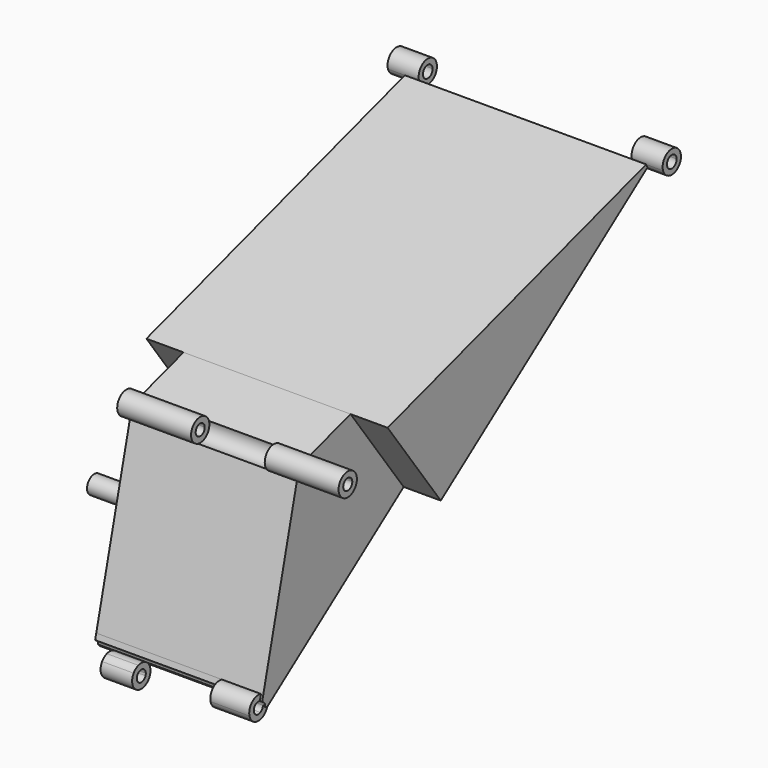
from build123d import *
from build123d import SkipClean  # not in build123d's __all__

# Parameters (mm, degrees)
F1_START = -16.65
F1_DEPTH = 79.6
F2_START = -37.25
F2_DEPTH = 34
F3_START = -114.75
F3_DEPTH = 33.5
F4_START = 62.75
F4_DEPTH = 79.6
F5_START = 45.55
F5_DEPTH = 42
F0_R     = 9.8
F6_DEPTH = 150
F8_DEPTH = 90
F9_DEPTH = 130


# Not quite as in the source:
# - after a boolean that leaves OpenCascade's solid faulty, fix() repairs it


with BuildPart() as f1:
    # F0 (on Right) → F1 (new body)
    with BuildSketch(Plane.YZ.offset(F1_START)):
        with BuildLine():
            Line((-18.1152243821, 20.3958344616), (-12.1555414908, 22.2498694633))
            ThreePointArc((-12.1555414908, 22.2498694633), (-32.9276080285, 27.0414189792), (-26.8836398395, 6.5986172255))
            Line((-26.8836398395, 6.5986172255), (-25.3948918397, 12.6598790865))
            ThreePointArc((-25.3948918397, 12.6598790865), (-28.3822482179, 22.7641569875), (-18.1152243821, 20.3958344616))
        make_face()
        with BuildLine():
            ThreePointArc((-26.8836398395, 6.5986172255), (-16.3247484731, 8.8719395429), (-11.5984598892, 18.5838074099))
            ThreePointArc((-11.5984598892, 18.5838074099), (-11.7385251038, 20.4378806886), (-12.1555414908, 22.2498694633))
            Line((-12.1555414908, 22.2498694633), (-18.1152243821, 20.3958344616))
            ThreePointArc((-18.1152243821, 20.3958344616), (-17.9091054013, 19.5002215043), (-17.8398752699, 18.5838074099))
            ThreePointArc((-17.8398752699, 18.5838074099), (-20.1759412293, 13.7835156961), (-25.3948918397, 12.6598790865))
            Line((-25.3948918397, 12.6598790865), (-26.8836398395, 6.5986172255))
        make_face()
    extrude(amount=-F1_DEPTH)



with BuildPart() as f2:
    # F0 (on Right) → F2 (new body)
    with BuildSketch(Plane.YZ.offset(F2_START)):
        with BuildLine():
            Line((-72.6551036638, -196.2316651642), (-67.6112595051, -192.5554031964))
            ThreePointArc((-67.6112595051, -192.5554031964), (-68.6065299554, -191.356834242), (-69.7448706932, -190.2932031158))
            ThreePointArc((-69.7448706932, -190.2932031158), (-70.6550390715, -193.4685207262), (-73.0869940433, -195.7038380233))
            ThreePointArc((-73.0869940433, -195.7038380233), (-72.8636664269, -195.9617109817), (-72.6551036638, -196.2316651642))
        make_face()
        with BuildLine():
            ThreePointArc((-69.7448706932, -190.2932031158), (-72.0550616531, -188.7913185641), (-74.6409019404, -187.8394417408))
            Line((-74.6409019404, -187.8394417408), (-76.1296499401, -193.9007036018))
            ThreePointArc((-76.1296499401, -193.9007036018), (-74.4747709929, -194.5769133854), (-73.0869940433, -195.7038380233))
            ThreePointArc((-73.0869940433, -195.7038380233), (-70.6550390715, -193.4685207262), (-69.7448706932, -190.2932031158))
        make_face()
        with BuildLine():
            Line((-76.1296499401, -193.9007036018), (-74.6409019404, -187.8394417408))
            ThreePointArc((-74.6409019404, -187.8394417408), (-78.1243753606, -187.4950233364), (-81.5644298108, -188.1425080744))
            ThreePointArc((-81.5644298108, -188.1425080744), (-81.831132306, -191.4349111758), (-80.3424675585, -194.3836271121))
            ThreePointArc((-80.3424675585, -194.3836271121), (-78.2793719358, -193.7643196914), (-76.1296499401, -193.9007036018))
        make_face()
        with BuildLine():
            ThreePointArc((-81.5644298108, -188.1425080744), (-85.124263165, -190.0540118898), (-87.8759224883, -193.012834513))
            ThreePointArc((-87.8759224883, -193.012834513), (-86.3429062121, -196.7512996317), (-83.6845909086, -199.7942620195))
            ThreePointArc((-83.6845909086, -199.7942620195), (-82.7744225302, -196.6189444092), (-80.3424675585, -194.3836271121))
            ThreePointArc((-80.3424675585, -194.3836271121), (-81.831132306, -191.4349111758), (-81.5644298108, -188.1425080744))
        make_face()
        with BuildLine():
            ThreePointArc((-83.6845909086, -199.7942620195), (-86.3429062121, -196.7512996317), (-87.8759224883, -193.012834513))
            ThreePointArc((-87.8759224883, -193.012834513), (-81.1414817132, -211.6423981781), (-65.2432511293, -199.8246319252))
            ThreePointArc((-65.2432511293, -199.8246319252), (-65.3210684593, -198.4409063564), (-65.5535391134, -197.0746306224))
            ThreePointArc((-65.5535391134, -197.0746306224), (-68.3051984367, -200.0334532455), (-71.865031791, -201.944957061))
            ThreePointArc((-71.865031791, -201.944957061), (-78.6766955162, -205.8260878027), (-83.6845909086, -199.7942620195))
        make_face()
        with BuildLine():
            ThreePointArc((-65.5535391134, -197.0746306224), (-66.3527593839, -194.7104559496), (-67.6112595051, -192.5554031964))
            Line((-67.6112595051, -192.5554031964), (-72.6551036638, -196.2316651642))
            ThreePointArc((-72.6551036638, -196.2316651642), (-71.7846521409, -197.9352316714), (-71.48466651, -199.8246319252))
            ThreePointArc((-71.48466651, -199.8246319252), (-71.5805107914, -200.9017178582), (-71.865031791, -201.944957061))
            ThreePointArc((-71.865031791, -201.944957061), (-68.3051984367, -200.0334532455), (-65.5535391134, -197.0746306224))
        make_face()
    extrude(amount=-F2_DEPTH)


with BuildPart() as f3:
    # F0 (on Right) → F3 (new body)
    with BuildSketch(Plane.YZ.offset(F3_START)):
        with BuildLine():
            Line((399.0634596914, 150.1785588691), (393.4857211205, 148.4433453134))
            ThreePointArc((393.4857211205, 148.4433453134), (394.2430188732, 146.5672949475), (395.2966478948, 144.840178638))
            Line((395.2966478948, 144.840178638), (400.0172420308, 148.2808362281))
            ThreePointArc((400.0172420308, 148.2808362281), (399.4623147045, 149.1904771133), (399.0634596914, 150.1785588691))
        make_face()
        with BuildLine():
            ThreePointArc((417.6114702803, 152.1094073668), (403.415981621, 164.3107575329), (393.4857211205, 148.4433453134))
            Line((393.4857211205, 148.4433453134), (399.0634596914, 150.1785588691))
            ThreePointArc((399.0634596914, 150.1785588691), (404.2935480778, 158.5356375547), (411.7700548997, 152.1094073668))
            ThreePointArc((411.7700548997, 152.1094073668), (407.2833502521, 145.9290641867), (400.0172420308, 148.2808362281))
            Line((400.0172420308, 148.2808362281), (395.2966478948, 144.840178638))
            ThreePointArc((395.2966478948, 144.840178638), (409.0926570886, 140.3749177698), (417.6114702803, 152.1094073668))
        make_face()
    extrude(amount=-F3_DEPTH)


with BuildPart() as f4:
    # F0 (on Right) → F4 (new body)
    with BuildSketch(Plane.YZ.offset(F4_START)):
        with BuildLine():
            Line((-18.1152243821, 20.3958344616), (-12.1555414908, 22.2498694633))
            ThreePointArc((-12.1555414908, 22.2498694633), (-32.9276080285, 27.0414189792), (-26.8836398395, 6.5986172255))
            Line((-26.8836398395, 6.5986172255), (-25.3948918397, 12.6598790865))
            ThreePointArc((-25.3948918397, 12.6598790865), (-28.3822482179, 22.7641569875), (-18.1152243821, 20.3958344616))
        make_face()
        with BuildLine():
            ThreePointArc((-26.8836398395, 6.5986172255), (-16.3247484731, 8.8719395429), (-11.5984598892, 18.5838074099))
            ThreePointArc((-11.5984598892, 18.5838074099), (-11.7385251038, 20.4378806886), (-12.1555414908, 22.2498694633))
            Line((-12.1555414908, 22.2498694633), (-18.1152243821, 20.3958344616))
            ThreePointArc((-18.1152243821, 20.3958344616), (-17.9091054013, 19.5002215043), (-17.8398752699, 18.5838074099))
            ThreePointArc((-17.8398752699, 18.5838074099), (-20.1759412293, 13.7835156961), (-25.3948918397, 12.6598790865))
            Line((-25.3948918397, 12.6598790865), (-26.8836398395, 6.5986172255))
        make_face()
    extrude(amount=F4_DEPTH)


with BuildPart() as f5:
    # F0 (on Right) → F5 (new body)
    with BuildSketch(Plane.YZ.offset(F5_START)):
        with BuildLine():
            ThreePointArc((-65.5535391134, -197.0746306224), (-66.3527593839, -194.7104559496), (-67.6112595051, -192.5554031964))
            Line((-67.6112595051, -192.5554031964), (-72.6551036638, -196.2316651642))
            ThreePointArc((-72.6551036638, -196.2316651642), (-71.7846521409, -197.9352316714), (-71.48466651, -199.8246319252))
            ThreePointArc((-71.48466651, -199.8246319252), (-71.5805107914, -200.9017178582), (-71.865031791, -201.944957061))
            ThreePointArc((-71.865031791, -201.944957061), (-68.3051984367, -200.0334532455), (-65.5535391134, -197.0746306224))
        make_face()
        with BuildLine():
            Line((-72.6551036638, -196.2316651642), (-67.6112595051, -192.5554031964))
            ThreePointArc((-67.6112595051, -192.5554031964), (-68.6065299554, -191.356834242), (-69.7448706932, -190.2932031158))
            ThreePointArc((-69.7448706932, -190.2932031158), (-70.6550390715, -193.4685207262), (-73.0869940433, -195.7038380233))
            ThreePointArc((-73.0869940433, -195.7038380233), (-72.8636664269, -195.9617109817), (-72.6551036638, -196.2316651642))
        make_face()
        with BuildLine():
            ThreePointArc((-63.5033797112, -190.2628332101), (-63.5081721417, -189.9189323753), (-63.5225457113, -189.5752986283))
            Line((-63.5225457113, -189.5752986283), (-67.6112595051, -192.5554031964))
            ThreePointArc((-67.6112595051, -192.5554031964), (-66.3527593839, -194.7104559496), (-65.5535391134, -197.0746306224))
            ThreePointArc((-65.5535391134, -197.0746306224), (-64.0270288389, -193.8196484134), (-63.5033797112, -190.2628332101))
        make_face()
        with BuildLine():
            ThreePointArc((-63.5225457113, -189.5752986283), (-66.1627938734, -182.6097693789), (-72.3303718412, -178.4323910032))
            Line((-72.3303718412, -178.4323910032), (-73.8225887621, -184.5077761678))
            ThreePointArc((-73.8225887621, -184.5077761678), (-70.8675740493, -186.7361817254), (-69.7447950918, -190.2628332101))
            ThreePointArc((-69.7447950918, -190.2628332101), (-69.7448139922, -190.27801821), (-69.7448706932, -190.2932031158))
            ThreePointArc((-69.7448706932, -190.2932031158), (-68.6065299554, -191.356834242), (-67.6112595051, -192.5554031964))
            Line((-67.6112595051, -192.5554031964), (-63.5225457113, -189.5752986283))
        make_face()
        with BuildLine():
            Line((-73.8225887621, -184.5077761678), (-72.3303718412, -178.4323910032))
            ThreePointArc((-72.3303718412, -178.4323910032), (-84.2875964997, -181.261186806), (-87.8759224883, -193.012834513))
            ThreePointArc((-87.8759224883, -193.012834513), (-85.124263165, -190.0540118898), (-81.5644298108, -188.1425080744))
            ThreePointArc((-81.5644298108, -188.1425080744), (-78.4371999949, -184.7411091299), (-73.8225887621, -184.5077761678))
        make_face()
        with BuildLine():
            ThreePointArc((-81.5644298108, -188.1425080744), (-85.124263165, -190.0540118898), (-87.8759224883, -193.012834513))
            ThreePointArc((-87.8759224883, -193.012834513), (-86.3429062121, -196.7512996317), (-83.6845909086, -199.7942620195))
            ThreePointArc((-83.6845909086, -199.7942620195), (-82.7744225302, -196.6189444092), (-80.3424675585, -194.3836271121))
            ThreePointArc((-80.3424675585, -194.3836271121), (-81.831132306, -191.4349111758), (-81.5644298108, -188.1425080744))
        make_face()
        with BuildLine():
            ThreePointArc((-80.3424675585, -194.3836271121), (-82.7744225302, -196.6189444092), (-83.6845909086, -199.7942620195))
            ThreePointArc((-83.6845909086, -199.7942620195), (-78.0541694481, -202.4048758122), (-71.865031791, -201.944957061))
            ThreePointArc((-71.865031791, -201.944957061), (-71.5805107914, -200.9017178582), (-71.48466651, -199.8246319252))
            ThreePointArc((-71.48466651, -199.8246319252), (-71.7846521409, -197.9352316714), (-72.6551036638, -196.2316651642))
            Line((-72.6551036638, -196.2316651642), (-77.58466651, -199.8246319252))
            Line((-77.58466651, -199.8246319252), (-76.7189272385, -196.2998766082))
            ThreePointArc((-76.7189272385, -196.2998766082), (-78.6964742873, -195.6552283891), (-80.3424675585, -194.3836271121))
        make_face()
        with BuildLine():
            Line((-77.58466651, -199.8246319252), (-72.6551036638, -196.2316651642))
            ThreePointArc((-72.6551036638, -196.2316651642), (-72.8636664269, -195.9617109817), (-73.0869940433, -195.7038380233))
            ThreePointArc((-73.0869940433, -195.7038380233), (-74.8569349642, -196.2823126202), (-76.7189272385, -196.2998766082))
            Line((-76.7189272385, -196.2998766082), (-77.58466651, -199.8246319252))
        make_face()
    extrude(amount=F5_DEPTH)


with BuildPart() as f6:
    # F0 (on Right) → F6 (new body)
    with BuildSketch(Plane.YZ):
        with Locations((0.0366982566, -86.2082434429)):
            Circle(F0_R)
    extrude(amount=-F6_DEPTH)


with BuildPart() as f7_1:
    # F7: instance of F3
    add(f3.part.mirror(Plane.YZ), clean=False)


with BuildPart() as f1_1:
    add(f1.part, clean=False)

    with SkipClean():  # cleaning this boolean's faces spoils the solid; the shape is the same uncleaned
        add(f2.part)  # F8 merges F2

    with SkipClean():  # cleaning this boolean's faces spoils the solid; the shape is the same uncleaned
        add(f4.part)  # F8 merges F4

    with SkipClean():  # cleaning this boolean's faces spoils the solid; the shape is the same uncleaned
        add(f5.part)  # F8 merges F5

    with SkipClean():  # cleaning this boolean's faces spoils the solid; the shape is the same uncleaned
        add(f6.part)  # F8 merges F6
    # F0 (on Right) → F8 (join, symmetric)
    with BuildSketch(Plane.YZ):
        with BuildLine():
            ThreePointArc((-12.1555414908, 22.2498694633), (-11.7385251038, 20.4378806886), (-11.5984598892, 18.5838074099))
            ThreePointArc((-11.5984598892, 18.5838074099), (-16.3247484731, 8.8719395429), (-26.8836398395, 6.5986172255))
            Line((-26.8836398395, 6.5986172255), (-72.3303718412, -178.4323910032))
            ThreePointArc((-72.3303718412, -178.4323910032), (-66.1627938734, -182.6097693789), (-63.5225457113, -189.5752986283))
            Line((-63.5225457113, -189.5752986283), (116.8328210509, -58.1212816783))
            Line((116.8328210509, -58.1212816783), (45.2393521867, 40.1052056848))
            Line((45.2393521867, 40.1052056848), (-12.1555414908, 22.2498694633))
        make_face()
        with Locations((0.0366982566, -86.2082434429)):
            Circle(F0_R, mode=Mode.SUBTRACT)
        with Locations((0.0366982566, -86.2082434429)):
            Circle(F0_R)
        with BuildLine():
            ThreePointArc((-63.5225457113, -189.5752986283), (-66.1627938734, -182.6097693789), (-72.3303718412, -178.4323910032))
            Line((-72.3303718412, -178.4323910032), (-73.8225887621, -184.5077761678))
            ThreePointArc((-73.8225887621, -184.5077761678), (-70.8675740493, -186.7361817254), (-69.7447950918, -190.2628332101))
            ThreePointArc((-69.7447950918, -190.2628332101), (-69.7448139922, -190.27801821), (-69.7448706932, -190.2932031158))
            ThreePointArc((-69.7448706932, -190.2932031158), (-68.6065299554, -191.356834242), (-67.6112595051, -192.5554031964))
            Line((-67.6112595051, -192.5554031964), (-63.5225457113, -189.5752986283))
        make_face()
    with SkipClean():  # cleaning this boolean's faces spoils the solid; the shape is the same uncleaned
        extrude(amount=F8_DEPTH, both=True)


    add(f3.part)  # F9 merges F3

    add(f7_1.part)  # F9 merges F7_1
    # F0 (on Right) → F9 (join, symmetric)
    with BuildSketch(Plane.YZ):
        with BuildLine():
            Line((393.4857211205, 148.4433453134), (45.2393521867, 40.1052056848))
            Line((45.2393521867, 40.1052056848), (116.8328210509, -58.1212816783))
            Line((116.8328210509, -58.1212816783), (395.2966478948, 144.840178638))
            ThreePointArc((395.2966478948, 144.840178638), (394.2430188732, 146.5672949475), (393.4857211205, 148.4433453134))
        make_face()
    extrude(amount=F9_DEPTH, both=True)

    add(f1_1.part.fix(), mode=Mode.REPLACE)


solid = f1_1.part
